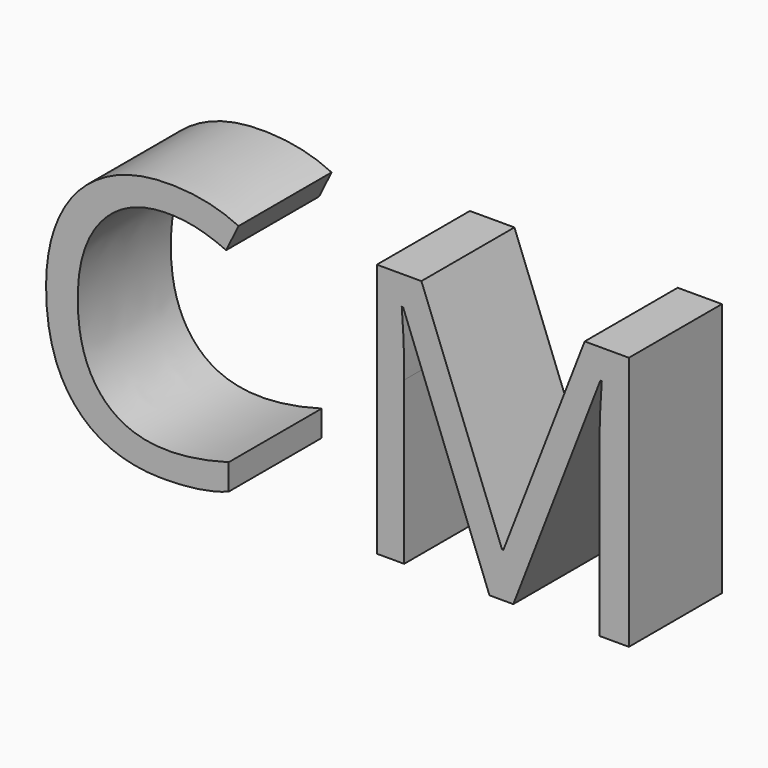
from build123d import *

# Parameters (mm, degrees)
F0_TEXT_SIZE = 77.8750050813
F1_DEPTH     = 25.4


# Not quite as in the source:
# - Text() gives the source's letters only with a copy of the font that has no kerning and outlines rounded to 1/6400 em; it was checked with that copy


with BuildPart() as f1:
    # F0 (on Front) → F1 (new body)
    with BuildSketch(Plane.XZ):
        with Locations((0, 0)):
            Text('C M', F0_TEXT_SIZE, font='Open Sans', text_align=(TextAlign.LEFT, TextAlign.BOTTOM))
    extrude(amount=F1_DEPTH)


solid = f1.part
